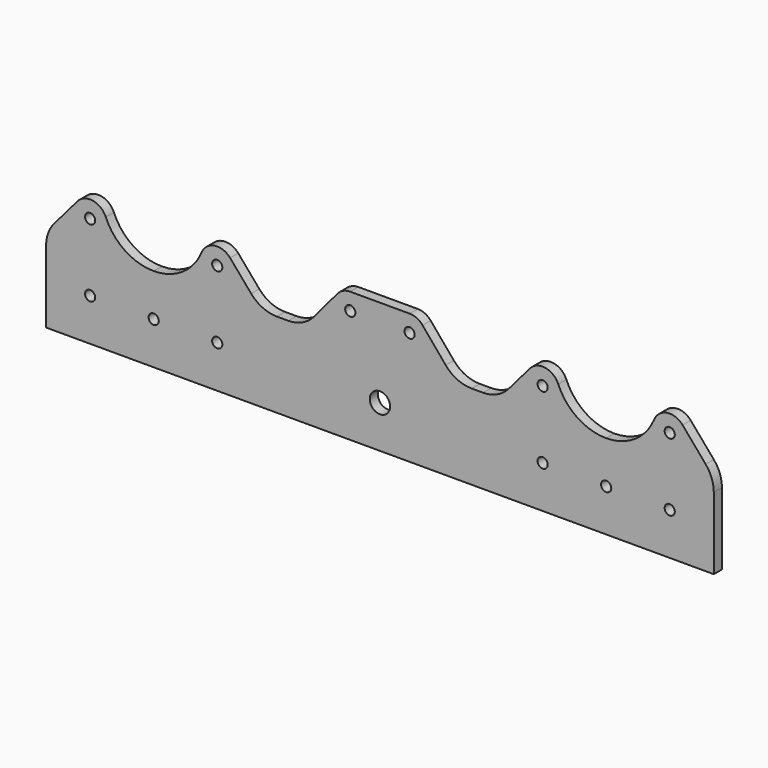
from build123d import *

# Parameters (mm, degrees)
F0_R     = 1.5
F0_R_2   = 3
F1_DEPTH = 3
F2_R     = 10


# Not quite as in the source:
# - a feature names something its author has since deleted; it is built from what else it names


with BuildPart() as f1:
    # F0 (on Front) → F1 (new body)
    with BuildSketch(Plane.XZ):
        Polygon((-197, 0), (0, 0), (0, 25), (-31.75, 25), (-63.5, 25), (-76.0906166883, 25), (-120.9093833117, 25), (-133.5, 25), (-165.25, 25), (-197, 25), align=None)
        with Locations((-184, 12.5)):
            Circle(F0_R, mode=Mode.SUBTRACT)
        with Locations((-165.25, 12.5)):
            Circle(F0_R, mode=Mode.SUBTRACT)
        with Locations((-146.5, 12.5)):
            Circle(F0_R, mode=Mode.SUBTRACT)
        with Locations((-98.5, 12.5)):
            Circle(F0_R_2, mode=Mode.SUBTRACT)
        with Locations((-50.5, 12.5)):
            Circle(F0_R, mode=Mode.SUBTRACT)
        with Locations((-31.75, 12.5)):
            Circle(F0_R, mode=Mode.SUBTRACT)
        with Locations((-13, 12.5)):
            Circle(F0_R, mode=Mode.SUBTRACT)
        with BuildLine():
            Line((-63.5, 25), (-31.75, 25))
            ThreePointArc((-31.75, 25), (-40.2438467547, 27.571729868), (-45.8846153846, 34.4230769231))
            ThreePointArc((-45.8846153846, 34.4230769231), (-49.720477364, 37.4388606439), (-54.2987189286, 35.7511128097))
            Line((-54.2987189286, 35.7511128097), (-63.5, 25))
        make_face()
        with Locations((-50.5, 32.5)):
            Circle(F0_R, mode=Mode.SUBTRACT)
        with BuildLine():
            Line((-31.75, 25), (0, 25))
            Line((0, 25), (-9.2012810714, 35.7511128097))
            ThreePointArc((-9.2012810714, 35.7511128097), (-13.779522636, 37.4388606439), (-17.6153846154, 34.4230769231))
            ThreePointArc((-17.6153846154, 34.4230769231), (-23.2561532453, 27.571729868), (-31.75, 25))
        make_face()
        with Locations((-13, 32.5)):
            Circle(F0_R, mode=Mode.SUBTRACT)
        with BuildLine():
            Line((-187.7987189286, 35.7511128097), (-197, 25))
            Line((-197, 25), (-165.25, 25))
            ThreePointArc((-165.25, 25), (-173.7438467547, 27.571729868), (-179.3846153846, 34.4230769231))
            ThreePointArc((-179.3846153846, 34.4230769231), (-183.220477364, 37.4388606439), (-187.7987189286, 35.7511128097))
        make_face()
        with Locations((-184, 32.5)):
            Circle(F0_R, mode=Mode.SUBTRACT)
        with BuildLine():
            ThreePointArc((-151.1153846154, 34.4230769231), (-156.7561532453, 27.571729868), (-165.25, 25))
            Line((-165.25, 25), (-133.5, 25))
            Line((-133.5, 25), (-142.7012810714, 35.7511128097))
            ThreePointArc((-142.7012810714, 35.7511128097), (-147.279522636, 37.4388606439), (-151.1153846154, 34.4230769231))
        make_face()
        with Locations((-146.5, 32.5)):
            Circle(F0_R, mode=Mode.SUBTRACT)
        with BuildLine():
            Line((-120.9093833117, 25), (-76.0906166883, 25))
            Line((-76.0906166883, 25), (-85.9197777844, 36.7139380484))
            ThreePointArc((-85.9197777844, 36.7139380484), (-87.6369086913, 38.0315389352), (-89.75, 38.5))
            Line((-89.75, 38.5), (-107.25, 38.5))
            ThreePointArc((-107.25, 38.5), (-109.3630913087, 38.0315389352), (-111.0802222156, 36.7139380484))
            Line((-111.0802222156, 36.7139380484), (-120.9093833117, 25))
        make_face()
        with Locations((-107.25, 33.5)):
            Circle(F0_R, mode=Mode.SUBTRACT)
        with Locations((-89.75, 33.5)):
            Circle(F0_R, mode=Mode.SUBTRACT)
    extrude(amount=F1_DEPTH)

    # F2
    f2_edges = [f1.edges().sort_by_distance(p)[0] for p in [
        (0, -1.5, 25),
        (-197, -1.5, 25),
        (-133.5, -1.5, 25),
        (-63.5, -1.5, 25),
        (-120.909383, -1.5, 25),
        (-76.090617, -1.5, 25),
    ]]
    fillet(f2_edges, radius=F2_R)


solid = f1.part
